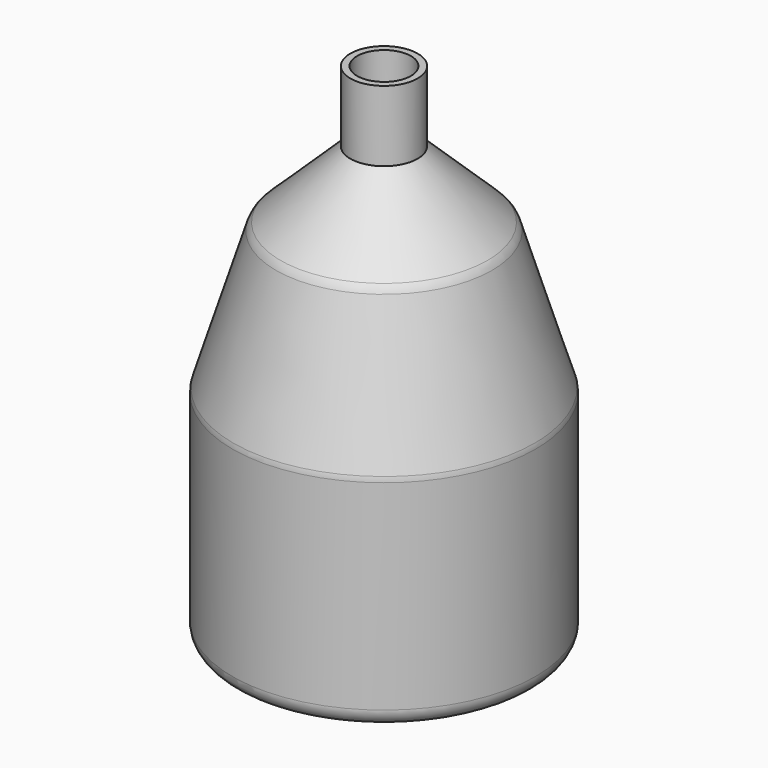
from build123d import *

# Parameters (mm, degrees)
F2_R = 5.08
F3_R = 5.08
F4_T = -2


with BuildPart() as f1:
    # F0 (on Front) → F1 (revolve)
    with BuildSketch(Plane.XZ):
        Polygon((0, 150), (0, 0), (45, 0), (45, 65.276236894), (31.6620995219, 108.2541429718), (10, 129.0087435294), (10, 150), align=None)
    revolve(axis=Axis((0, 0, 75), (0, 0, -1)))

    # F2
    f2_edges = [f1.edges().sort_by_distance(p)[0] for p in [
        (-45, 0, 0),
        (-45, 0, 65.276237),
        (45, 0, 32.638118),
    ]]
    fillet(f2_edges, radius=F2_R)

    # F3
    f3_edges = [f1.edges().sort_by_distance(p)[0] for p in [
        (-31.6621, 0, 108.254143),
    ]]
    fillet(f3_edges, radius=F3_R)

    # F4
    f4_openings = [f1.faces().sort_by_distance(p)[0] for p in [
        (0, 0, 150),
    ]]
    offset(amount=F4_T, openings=f4_openings, kind=Kind.INTERSECTION)


solid = f1.part
